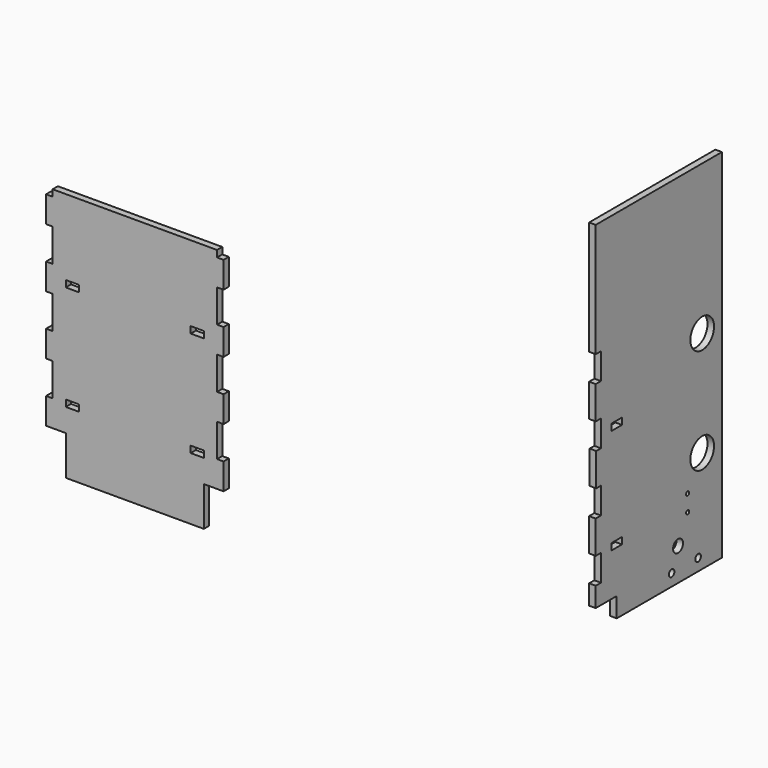
from build123d import *

# Parameters (mm, degrees)
F0_W      = 6.35
F0_H      = 25.4
F0_H_2    = 6.35
F1_DEPTH  = 6.35
F2_W      = 5.7369639019
F2_H      = 31.75
F2_W_2    = 6.35
F2_H_2    = 19.05
F2_H_3    = 103.632
F2_H_4    = 6.35
F3_DEPTH  = 6.35
F4_R      = 14.2875
F5_DEPTH  = 6.35
F6_W      = 12.7
F6_H      = 6.35
F7_DEPTH  = 6.35
F8_W      = 12.7
F8_H      = 6.35
F9_DEPTH  = 6.35
F11_DEPTH = 6.35
F12_R     = 6
F13_DEPTH = 25.4
F14_R     = 3.3782
F14_R_2   = 1.905
F15_DEPTH = 6.35


# Not quite as in the source:
# - a feature names something its author has since deleted; it is built from what else it names


with BuildPart() as f1:
    # F0 (on Front) → F1 (new body)
    with BuildSketch(Plane.XZ):
        with Locations((-498.5113858938, -21.1435346045)):
            Rectangle(F0_W, F0_H)
        with Locations((-498.5113858938, -78.2935346045)):
            Rectangle(F0_W, F0_H)
        with Locations((-498.5113858938, -135.4435346045)):
            Rectangle(F0_W, F0_H)
        with Locations((-498.5113858938, -192.5935346045)):
            Rectangle(F0_W, F0_H)
        with Locations((-498.5113858938, -240.2185346045)):
            Rectangle(F0_W, F0_H_2)
        with Locations((-333.4113858938, -240.2185346045)):
            Rectangle(F0_W, F0_H_2)
        with Locations((-333.4113858938, -192.5935346045)):
            Rectangle(F0_W, F0_H)
        with Locations((-333.4113858938, -135.4435346045)):
            Rectangle(F0_W, F0_H)
        with Locations((-333.4113858938, -78.2935346045)):
            Rectangle(F0_W, F0_H)
        with Locations((-333.4113858938, -21.1435346045)):
            Rectangle(F0_W, F0_H)
        Polygon((-495.3363858938, -237.0435346045), (-495.3363858938, -243.3935346045), (-336.5863858938, -243.3935346045), (-336.5863858938, -237.0435346045), (-336.5863858938, -205.2935346045), (-336.5863858938, -179.8935346045), (-336.5863858938, -148.1435346045), (-336.5863858938, -122.7435346045), (-336.5863858938, -90.9935346045), (-336.5863858938, -65.5935346045), (-336.5863858938, -33.8435346045), (-336.5863858938, -8.4435346045), (-336.5863858938, -2.0935346045), (-495.3363858938, -2.0935346045), (-495.3363858938, -8.4435346045), (-495.3363858938, -33.8435346045), (-495.3363858938, -65.5935346045), (-495.3363858938, -90.9935346045), (-495.3363858938, -122.7435346045), (-495.3363858938, -148.1435346045), (-495.3363858938, -179.8935346045), (-495.3363858938, -205.2935346045), align=None)
    extrude(amount=F1_DEPTH)

    # F8 (on face) → F9 (cut)
    with BuildSketch(Plane.XZ.offset(6.35)):
        with Locations((-476.2863858938, -78.2935346045)):
            Rectangle(F8_W, F8_H)
        with Locations((-476.2863858938, -179.8935346045)):
            Rectangle(F8_W, F8_H)
        with Locations((-355.6363858938, -78.2935346045)):
            Rectangle(F8_W, F8_H)
        with Locations((-355.6363858938, -179.8935346045)):
            Rectangle(F8_W, F8_H)
    extrude(amount=-F9_DEPTH, mode=Mode.SUBTRACT)

    # F10 (on face) → F11 (cut)
    with BuildSketch(Plane.XZ.offset(6.35)):
        Polygon((-501.6863858938, -243.3935346045), (-482.6363858938, -243.3935346045), (-482.6363858938, -205.2935346045), (-495.3363858938, -205.2935346045), (-495.3363858938, -237.0435346045), (-501.6863858938, -237.0435346045), align=None)
        Polygon((-349.2863858938, -205.2935346045), (-349.2863858938, -243.3935346045), (-330.2363858938, -243.3935346045), (-330.2363858938, -237.0435346045), (-336.5863858938, -237.0435346045), (-336.5863858938, -205.2935346045), align=None)
    extrude(amount=-F11_DEPTH, mode=Mode.SUBTRACT)


with BuildPart() as f3:
    # F2 (on Right) → F3 (new body)
    with BuildSketch(Plane.YZ):
        with Locations((25.6664895297, -89.2577976048)):
            Rectangle(F2_W, F2_H)
        with Locations((25.3599714807, -32.1077976048)):
            Rectangle(F2_W_2, F2_H)
        with Locations((25.3599714807, -146.4077976048)):
            Rectangle(F2_W_2, F2_H)
        with Locations((25.3599714807, -197.2077976048)):
            Rectangle(F2_W_2, F2_H_2)
        with Locations((25.3599714807, 67.3332023952)):
            Rectangle(F2_W_2, F2_H_3)
        with Locations((25.3599714807, 12.3422023952)):
            Rectangle(F2_W_2, F2_H_4)
        Polygon((28.5349714807, 9.1672023952), (28.5349714807, -16.2327976048), (28.5349714807, -47.9827976048), (28.5349714807, -73.3827976048), (28.5349714807, -105.1327976048), (28.5349714807, -130.5327976048), (28.5349714807, -162.2827976048), (28.5349714807, -187.6827976048), (28.5349714807, -206.7327976048), (47.5849714807, -206.7327976048), (47.5849714807, -225.7827976048), (174.5849714807, -225.7827976048), (174.5849714807, 119.1492023952), (28.5349714807, 119.1492023952), (28.5349714807, 15.5172023952), align=None)
    extrude(amount=F3_DEPTH)

    # F4 (on face) → F5 (cut)
    with BuildSketch(Plane(origin=(0, 0, 0), x_dir=(0, -1, 0), z_dir=(-1, 0, 0))):
        with Locations((-150.7724714807, -25.3259976048)):
            Circle(F4_R)
        with Locations((-150.7724714807, -126.9259976048)):
            Circle(F4_R)
    extrude(amount=-F5_DEPTH, mode=Mode.SUBTRACT)

    # F6 (on face) → F7 (cut)
    with BuildSketch(Plane(origin=(0, 0, 0), x_dir=(0, -1, 0), z_dir=(-1, 0, 0))):
        with Locations((-47.5849714807, -60.6827976048)):
            Rectangle(F6_W, F6_H)
        with Locations((-47.5849714807, -162.2827976048)):
            Rectangle(F6_W, F6_H)
    extrude(amount=-F7_DEPTH, mode=Mode.SUBTRACT)

    # F12 (on face) → F13 (cut)
    with BuildSketch(Plane(origin=(0, 0, 0), x_dir=(0, -1, 0), z_dir=(-1, 0, 0))):
        with Locations((-121.6259714807, -194.3121976048)):
            Circle(F12_R)
    extrude(amount=-F13_DEPTH, mode=Mode.SUBTRACT)

    # F14 (on face) → F15 (cut)
    with BuildSketch(Plane(origin=(0, 0, 0), x_dir=(0, -1, 0), z_dir=(-1, 0, 0))):
        with Locations((-145.8321714807, -214.2765976048)):
            Circle(F14_R)
        with Locations((-113.8281714807, -214.2765976048)):
            Circle(F14_R)
        with Locations((-133.2083714807, -170.3853976048)):
            Circle(F14_R_2)
        with Locations((-133.2083714807, -154.3833976048)):
            Circle(F14_R_2)
    extrude(amount=-F15_DEPTH, mode=Mode.SUBTRACT)


solid = Compound([f1.part, f3.part])
